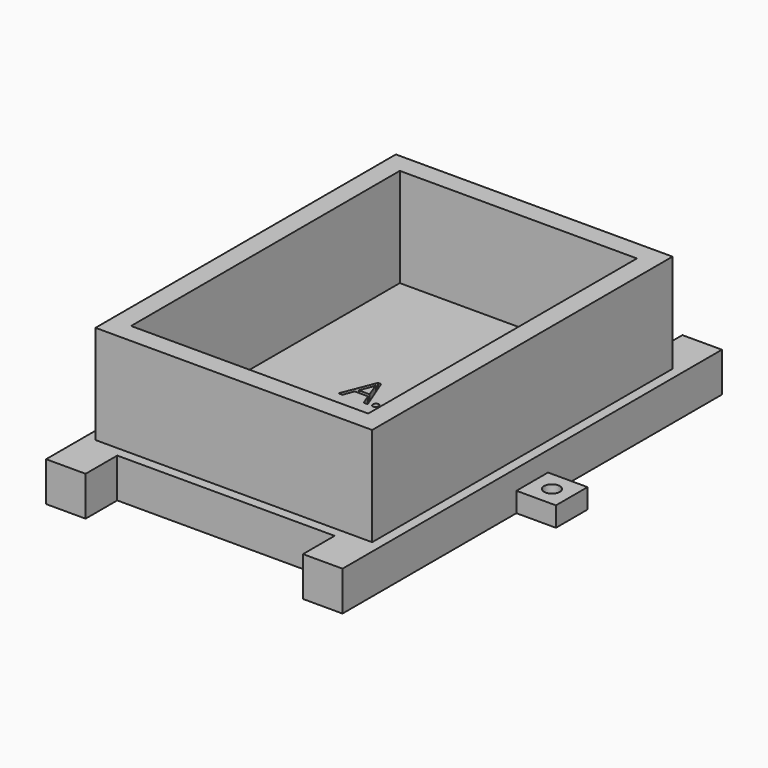
from build123d import *

# Parameters (mm, degrees)
F0_W          = 75
F0_H          = 100
F0_W_2        = 50
F0_H_2        = 75
F1_DEPTH      = 10
F2_W          = 70
F2_H          = 95
F2_W_2        = 60
F2_H_2        = 85
F3_DEPTH      = 25
F4_W          = 10
F4_H          = 10
F5_DEPTH      = 10
F6_W          = 10
F6_H          = 10
F7_DEPTH      = 10
F8_W          = 10
F8_H          = 5
F9_DEPTH      = 10
F10_R         = 2
F11_DEPTH     = 3
F12_TEXT_SIZE = 11.7033921551
F13_DEPTH     = 2


# Not quite as in the source:
# - a feature names something its author has since deleted; it is built from what else it names
# - Text() gives the source's letters only with a copy of the font that has no kerning and outlines rounded to 1/6400 em; it was checked with that copy


with BuildPart() as f1:
    # F0 (on Top) → F1 (new body)
    with BuildSketch(Plane.XY):
        with Locations((-57.8411258757, -74.6295199012)):
            Rectangle(F0_W, F0_H)
        with Locations((-57.8411258757, -74.6295199012)):
            Rectangle(F0_W_2, F0_H_2, mode=Mode.SUBTRACT)
        with Locations((-57.8411258757, -74.6295199012)):
            Rectangle(F0_W_2, F0_H_2)
    extrude(amount=F1_DEPTH)

    # F2 (on face) → F3 (join)
    with BuildSketch(Plane.XY.offset(10)):
        with Locations((-57.8411258757, -74.6295199012)):
            Rectangle(F2_W, F2_H)
        with Locations((-57.8411258757, -74.6295199012)):
            Rectangle(F2_W_2, F2_H_2, mode=Mode.SUBTRACT)
    extrude(amount=F3_DEPTH)

    # F4 (on face) → F5 (join)
    with BuildSketch(Plane.XZ.offset(124.6295199012)):
        with Locations((-25.3411258757, 5)):
            Rectangle(F4_W, F4_H)
        with Locations((-90.3411258757, 5)):
            Rectangle(F4_W, F4_H)
    extrude(amount=F5_DEPTH)

    # F6 (on face) → F7 (join)
    with BuildSketch(Plane(origin=(0, -24.6295199012, 0), x_dir=(-1, 0, 0), z_dir=(0, 1, 0))):
        with Locations((25.3411258757, 5)):
            Rectangle(F6_W, F6_H)
        with Locations((90.3411258757, 5)):
            Rectangle(F6_W, F6_H)
    extrude(amount=F7_DEPTH)

    # F8 (on face) → F9 (join)
    with BuildSketch(Plane.YZ.offset(-20.3411258757)):
        with Locations((-74.6295199012, 2.5)):
            Rectangle(F8_W, F8_H)
    extrude(amount=F9_DEPTH)

    # F10 (on face) → F11 (cut)
    with BuildSketch(Plane.XY.offset(5)):
        with Locations((-15.3411258757, -74.6295199012)):
            Circle(F10_R)
    extrude(amount=-F11_DEPTH, mode=Mode.SUBTRACT)

    # F12 (on face) → F13 (cut)
    with BuildSketch(Plane.XY.offset(10)):
        with Locations((-67.8411258757, -76.5559622529)):
            Text('A.T.', F12_TEXT_SIZE, font='Open Sans', text_align=(TextAlign.LEFT, TextAlign.BOTTOM))
    extrude(amount=-F13_DEPTH, mode=Mode.SUBTRACT)


solid = f1.part
